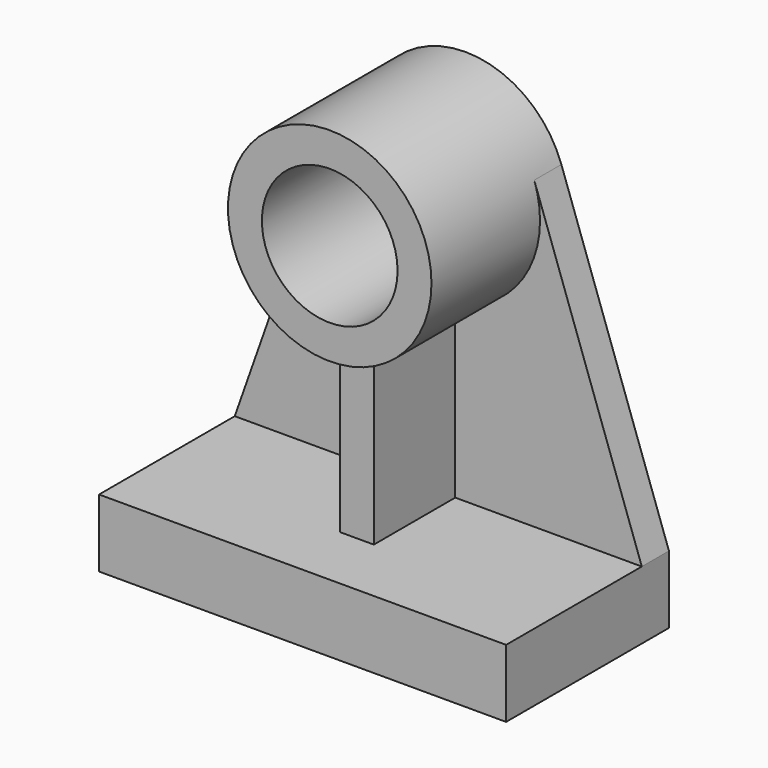
from build123d import *

# Parameters (mm, degrees)
F0_R     = 76.2
F0_R_2   = 50.8
F1_DEPTH = 127
F3_DEPTH = 25.4
F4_W     = 304.8
F4_H     = 50.8
F5_DEPTH = 152.4
F7_DEPTH = 76.2


with BuildPart() as f1:
    # F0 (on Front) → F1 (new body)
    with BuildSketch(Plane.XZ):
        Circle(F0_R)
        Circle(F0_R_2, mode=Mode.SUBTRACT)
    extrude(amount=F1_DEPTH)

    # F2 (on Front) → F3 (join)
    with BuildSketch(Plane.XZ):
        with BuildLine():
            ThreePointArc((71.8681337184, 25.3261002888), (75.1092264284, 12.8469492616), (76.2, 0))
            ThreePointArc((76.2, 0), (-12.8469492616, -75.1092264284), (-71.8681337184, 25.3261002888))
            Line((-71.8681337184, 25.3261002888), (-152.4, -203.2))
            Line((-152.4, -203.2), (152.4, -203.2))
            Line((152.4, -203.2), (71.8681337184, 25.3261002888))
        make_face()
    extrude(amount=F3_DEPTH)

    # F4 (on Front) → F5 (join)
    with BuildSketch(Plane.XZ):
        with Locations((0, -228.6)):
            Rectangle(F4_W, F4_H)
    extrude(amount=F5_DEPTH)

    # F6 (on face) → F7 (join)
    with BuildSketch(Plane.XZ.offset(25.4)):
        with BuildLine():
            Line((-12.7, -75.1342132454), (-12.7, -203.2))
            Line((-12.7, -203.2), (12.7, -203.2))
            Line((12.7, -203.2), (12.7, -75.1342132454))
            ThreePointArc((12.7, -75.1342132454), (0, -76.2), (-12.7, -75.1342132454))
        make_face()
    extrude(amount=F7_DEPTH)


with BuildPart() as f8_1:
    # F8: copy of F1
    add(f1.part)


solid = f1.part
